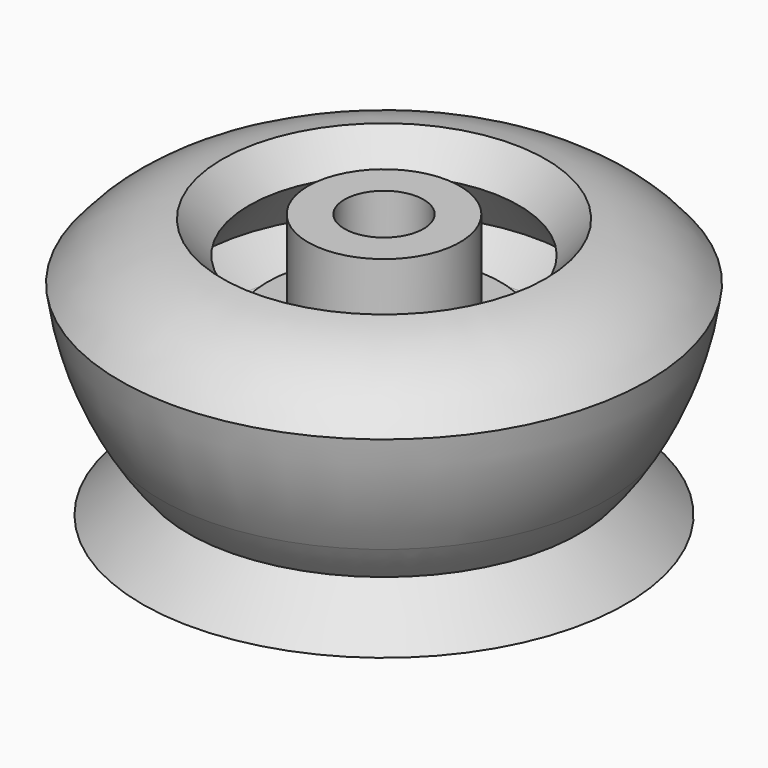
from build123d import *

# Parameters (mm, degrees)
F3_D     = 9.525
F3_DEPTH = 9.271
F3_TIP   = 2.8615986981
F4_R     = 1.5875
F5_DEPTH = 21.717
F6_R     = 2.54
F7_R     = 4.191


with BuildPart() as f1:
    # F0 (on Front) → F1 (revolve)
    with BuildSketch(Plane.XZ):
        with BuildLine():
            Line((0, -26.3518410662), (0, 0))
            Line((0, 0), (0, 11.7481589338))
            Line((0, 11.7481589338), (-9.1452337801, 11.7481589338))
            Line((-9.1452337801, 11.7481589338), (-9.1452337801, 0))
            Line((-9.1452337801, 0), (-14.0358982608, 0))
            Line((-14.0358982608, 0), (-16.0151850432, -6.9885868579))
            Line((-16.0151850432, -6.9885868579), (-22.680465132, 0))
            Line((-22.680465132, 0), (-16.2254925817, 7.4013243429))
            Line((-16.2254925817, 7.4013243429), (-19.4562915713, 11.250785552))
            ThreePointArc((-19.4562915713, 11.250785552), (-26.295058761, 9.081502601), (-31.75, 4.4212299399))
            ThreePointArc((-31.75, 4.4212299399), (-30.0167425827, -2.9230382279), (-26.851716639, -9.7732255955))
            ThreePointArc((-26.851716639, -9.7732255955), (-25.2807815933, -12.1832568025), (-23.5026830704, -14.4447724402))
            Line((-23.5026830704, -14.4447724402), (-29.0771815926, -20.0948305428))
            Line((-29.0771815926, -20.0948305428), (-21.4918367565, -21.9874773175))
            Line((-21.4918367565, -21.9874773175), (-11.1905843171, -23.3150029238))
            Line((-11.1905843171, -23.3150029238), (-7.8794877043, -23.0577233122))
            Line((-7.8794877043, -23.0577233122), (-3.175, -26.3518410662))
            Line((-3.175, -26.3518410662), (0, -26.3518410662))
        make_face()
    revolve(axis=Axis((0, 0, 5.8740794669), (0, 0, -1)))

    # F3
    with Locations(Plane.XY.offset(11.7481589338)):
        with Locations((0, 0)):
            Hole(F3_D / 2, depth=F3_DEPTH)
            with Locations((0, 0, -(F3_DEPTH + F3_TIP / 2))):  # 118° drill point
                Cone(0, F3_D / 2, F3_TIP, mode=Mode.SUBTRACT)

    # F4 (on face) → F5 (cut)
    with BuildSketch(Plane(origin=(0, 0, -26.3518410662), x_dir=(1, 0, 0), z_dir=(0, 0, -1))):
        Circle(F4_R)
    extrude(amount=-F5_DEPTH, mode=Mode.SUBTRACT)

    # F6
    f6_edges = [f1.edges().sort_by_distance(p)[0] for p in [
        (16.015185, 0, -6.988587),
    ]]
    fillet(f6_edges, radius=F6_R)

    # F7
    f7_edges = [f1.edges().sort_by_distance(p)[0] for p in [
        (7.879488, 0, -23.057723),
        (3.175, 0, -26.351841),
    ]]
    fillet(f7_edges, radius=F7_R)


solid = f1.part
